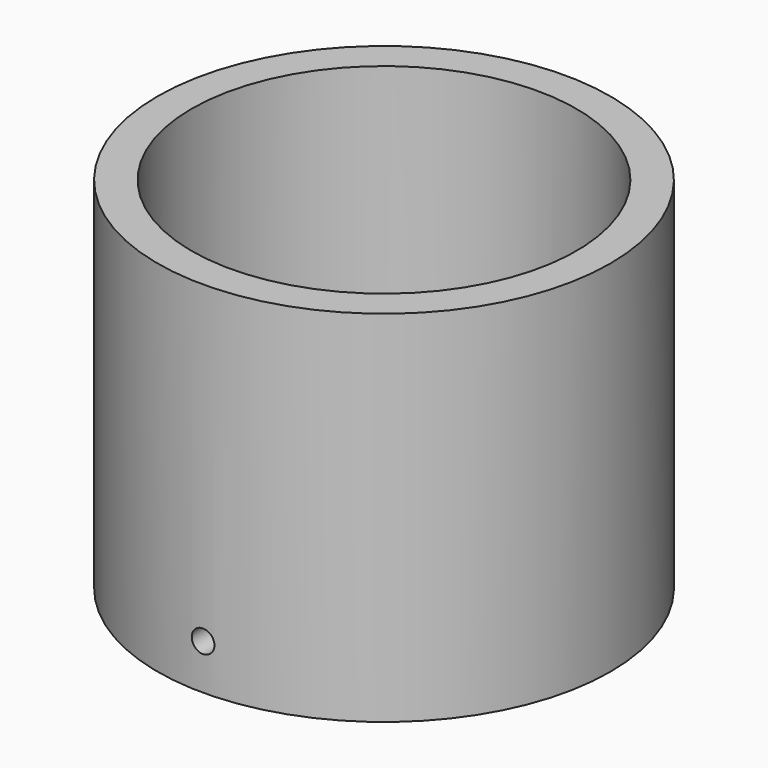
from build123d import *

# Parameters (mm, degrees)
F0_W     = 2.4
F0_H     = 25.4
F2_R     = 0.8
F3_DEPTH = 40


# Not quite as in the source:
# - a pattern or mirror of a feature is missing from the dataset's text; its kind, count and spacing are read off the source's solid


with BuildPart() as f1:
    # F0 (on Front) → F1 (revolve)
    with BuildSketch(Plane.XZ):
        with Locations((-14.8, 12.7)):
            Rectangle(F0_W, F0_H)
    revolve(axis=Axis((0, 0, -8.8682172461), (0, 0, -1)))

    # F2 (on Front) → F3 (cut)
    with BuildSketch(Plane.XZ):
        with Locations((0, 3.2)):
            Circle(F2_R)
    f3 = extrude(amount=F3_DEPTH, mode=Mode.SUBTRACT)

    # F3_copies: F3 across plane
    add(f3.mirror(Plane.ZX.offset(5e-06)), mode=Mode.SUBTRACT)


solid = f1.part
